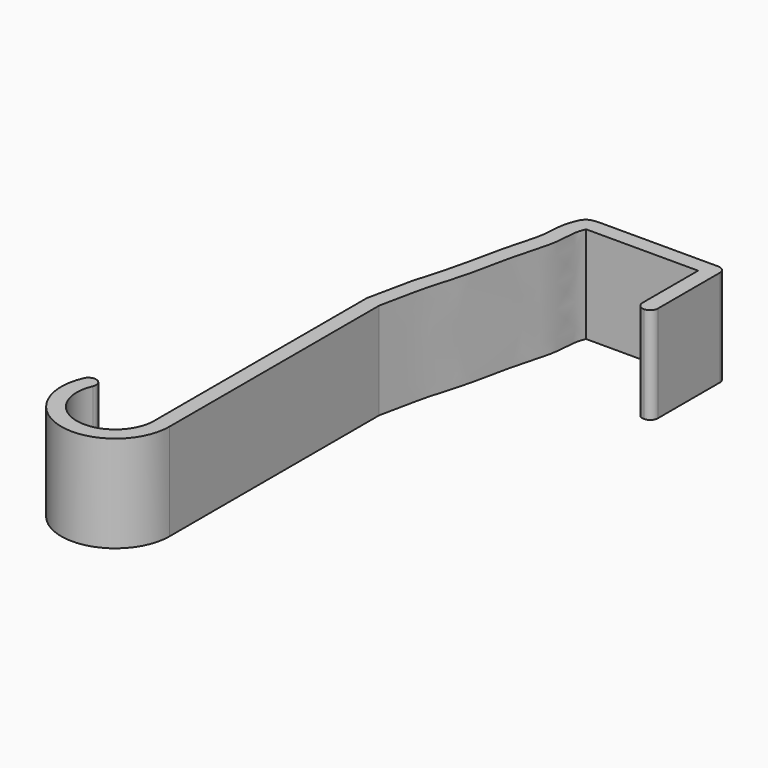
from build123d import *

# Parameters (mm, degrees)
F1_DEPTH = 25


# Not quite as in the source:
# - ends of sketch curves that miss each other by under 0.0002 mm in the source are joined
# - the dataset's text gives a spline's control points without its knots; the knots are read off the source's solid


with BuildPart() as f1:
    # F0 (on Top) → F1 (new body)
    with BuildSketch(Plane.XY):
        with BuildLine():
            add(Edge.make_bspline(
                [(-19.5588455008, 0), (-19.8547467578, -0.7587121148), (-20.5814890027, -2.6221045495), (-20.4762964436, -8.4124422113), (-23.0958469727, -16.4760646806), (-24.8049259302, -25.0087801975), (-26.4580974656, -32.6068882185), (-28.7441018372, -39.541057158), (-29.8720437239, -45.2853600599), (-30.7836047074, -49.8128469401), (-31.3333741179, -52.1760059191)],
                knots=[0, 0, 0, 0, 0.0793438206, 0.194937933, 0.3386430534, 0.4838589857, 0.6208280007, 0.7518942696, 0.8701646738, 1, 1, 1, 1], degree=3))
            Line((-19.5588455008, 0), (-19.5588455008, 4))
            add(Edge.make_bspline(
                [(-23.4054287408, 1.5001853718), (-22.4370600331, 3.753568072), (-21.5017963201, 3.7808972411), (-19.5588455008, 4)],
                knots=[0, 0, 0, 0, 4.5875130297, 4.5875130297, 4.5875130297, 4.5875130297], degree=3))
            add(Edge.make_bspline(
                [(-23.4054287408, 1.5001853718), (-23.5219691483, 1.2013673813), (-23.7293124168, 0.6738952667), (-24.0169631636, -0.2061714914), (-24.1843465416, -0.825964403), (-24.3019046559, -1.358925189), (-24.380557819, -1.7785205991), (-24.4461947396, -2.2070079291), (-24.4977412732, -2.6186937553), (-24.5397579334, -3.0227674809), (-24.5860639372, -3.5512825525), (-24.6493662091, -4.4556865012), (-24.7083870547, -5.4574567347), (-24.7901423209, -6.4309767835), (-24.8692520188, -7.145641856), (-24.9716503148, -7.8351414586), (-25.1109180769, -8.5793397575), (-25.2818640842, -9.3634854445), (-25.5474528739, -10.4597959218), (-25.8603268818, -11.6229235599), (-26.2001022802, -12.840590262), (-26.462885771, -13.7792534542), (-26.7277166993, -14.7399540771), (-26.9896680705, -15.7270131039), (-27.2371367385, -16.7097087789), (-27.5503163422, -18.0104976324), (-27.9139199917, -19.61727219), (-28.31747573, -21.505875167), (-28.6995058558, -23.3471136993), (-29.0706034762, -25.1297394304), (-29.4424747831, -26.8616484076), (-29.8238968076, -28.5486895759), (-30.1570356563, -29.9214268136), (-30.4373891243, -31.0044201468), (-30.7274039195, -32.0738312485), (-31.120874277, -33.4317377183), (-31.6188014703, -35.0851684996), (-32.0341010344, -36.472259808), (-32.3533128023, -37.5833315021), (-32.58346339, -38.4190840817), (-32.7982403771, -39.2488212516), (-33.0602849113, -40.3259366128), (-33.3522798393, -41.6358164684), (-33.6678537173, -43.1745499916), (-34.0735239246, -45.2233271681), (-34.6100121546, -47.8916302659), (-35.085574352, -50.0793596494), (-35.3333743001, -51.1483845336)],
                knots=[0, 0, 0, 0, 0.03125, 0.046875, 0.0625, 0.0703125, 0.078125, 0.0859375, 0.09375, 0.1015625, 0.109375, 0.125, 0.15625, 0.171875, 0.1875, 0.203125, 0.21875, 0.234375, 0.25, 0.28125, 0.296875, 0.3125, 0.328125, 0.34375, 0.359375, 0.375, 0.40625, 0.4375, 0.46875, 0.5, 0.53125, 0.5625, 0.59375, 0.609375, 0.625, 0.65625, 0.6875, 0.71875, 0.734375, 0.75, 0.765625, 0.78125, 0.8125, 0.84375, 0.875, 0.9375, 0.9982551796, 0.9982551796, 0.9982551796, 0.9982551796], degree=3))
            Line((-35.3333743001, -51.1483845336), (-35.3333741179, -120))
            ThreePointArc((-35.3333741179, -120), (-47.4390651757, -129.7757897466), (-54.4465871517, -115.8830413895))
            ThreePointArc((-54.4465871517, -115.8830413895), (-54.3456664022, -114.5120147393), (-55.1535808039, -113.3997317748))
            ThreePointArc((-55.1535808039, -113.3997317748), (-56.8168646866, -113.1360863112), (-58.0918723652, -114.2362579453))
            ThreePointArc((-58.0918723652, -114.2362579453), (-48.2813415988, -133.6861056452), (-31.3333741179, -120))
            Line((-31.3333741179, -120), (-31.3333741179, -52.1760059191))
        make_face()
        with BuildLine():
            Line((-19.5588455008, 0), (9.4411544992, 0))
            Line((9.4411544992, 0), (13.4411544992, 0))
            Line((13.4411544992, 0), (13.4411544992, 2))
            ThreePointArc((13.4411544992, 2), (12.8553680616, 3.4142135624), (11.4411544992, 4))
            Line((11.4411544992, 4), (-19.5588455008, 4))
            Line((-19.5588455008, 4), (-19.5588455008, 0))
        make_face()
        with BuildLine():
            Line((13.4411544992, 0), (9.4411544992, 0))
            Line((9.4411544992, 0), (9.4411544992, -18))
            ThreePointArc((9.4411544992, -18), (10.0269409368, -19.4142135624), (11.4411544992, -20))
            ThreePointArc((11.4411544992, -20), (12.8553680616, -19.4142135624), (13.4411544992, -18))
            Line((13.4411544992, -18), (13.4411544992, 0))
        make_face()
    extrude(amount=F1_DEPTH)


solid = f1.part
